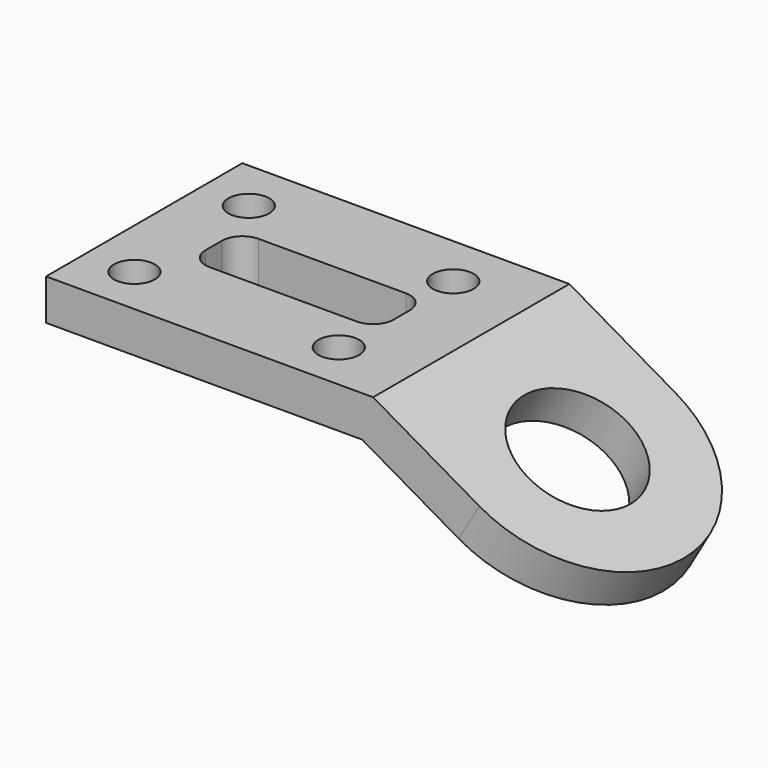
from build123d import *

# Parameters (mm, degrees)
F1_DEPTH = 60
F2_R     = 29.99999
F3_R     = 15
F4_DEPTH = 10
F5_R     = 5
F6_DEPTH = 10
F7_W     = 46
F7_H     = 15
F8_DEPTH = 10
F9_R     = 5
F10_R    = 5


# Not quite as in the source:
# - a fillet or chamfer is up to 0.001 mm smaller than in the source, because OpenCascade refuses the exact size


with BuildPart() as f1:
    # F0 (on Front) → F1 (new body)
    with BuildSketch(Plane.XZ):
        Polygon((80, 0), (0, 0), (0, -10), (77.3205080757, -10), (126.9615242271, -38.6602540378), (131.9615242271, -30), align=None)
    extrude(amount=F1_DEPTH)

    # F2 (radius 30 in the source; OpenCascade refuses exactly that, so slightly less here)
    f2_edges = [f1.edges().sort_by_distance(p)[0] for p in [
        (129.461524, 0, -34.330127),
        (129.461524, -60, -34.330127),
    ]]
    fillet(f2_edges, radius=F2_R)

    # F3 (on face) → F4 (cut, through all)
    with BuildSketch(Plane(origin=(20, 0, 34.6410161514), x_dir=(0.8660254038, 0, -0.5), z_dir=(0.5, 0, 0.8660254038))):
        with Locations((99.2820323028, -30)):
            Circle(F3_R)
    extrude(amount=-F4_DEPTH, mode=Mode.SUBTRACT)

    # F5 (on face) → F6 (cut, through all)
    with BuildSketch(Plane.XY):
        with Locations((12, -13)):
            Circle(F5_R)
        with Locations((12, -48)):
            Circle(F5_R)
        with Locations((62, -48)):
            Circle(F5_R)
        with Locations((62, -13)):
            Circle(F5_R)
    extrude(amount=-F6_DEPTH, mode=Mode.SUBTRACT)

    # F7 (on face) → F8 (cut, through all)
    with BuildSketch(Plane.XY):
        with Locations((40, -30)):
            Rectangle(F7_W, F7_H)
    extrude(amount=-F8_DEPTH, mode=Mode.SUBTRACT)

    # F9
    f9_edges = [f1.edges().sort_by_distance(p)[0] for p in [
        (17, -22.5, -5),
    ]]
    fillet(f9_edges, radius=F9_R)

    # F10
    f10_edges = [f1.edges().sort_by_distance(p)[0] for p in [
        (63, -22.5, -5),
        (63, -37.5, -5),
        (17, -37.5, -5),
    ]]
    fillet(f10_edges, radius=F10_R)


solid = f1.part
